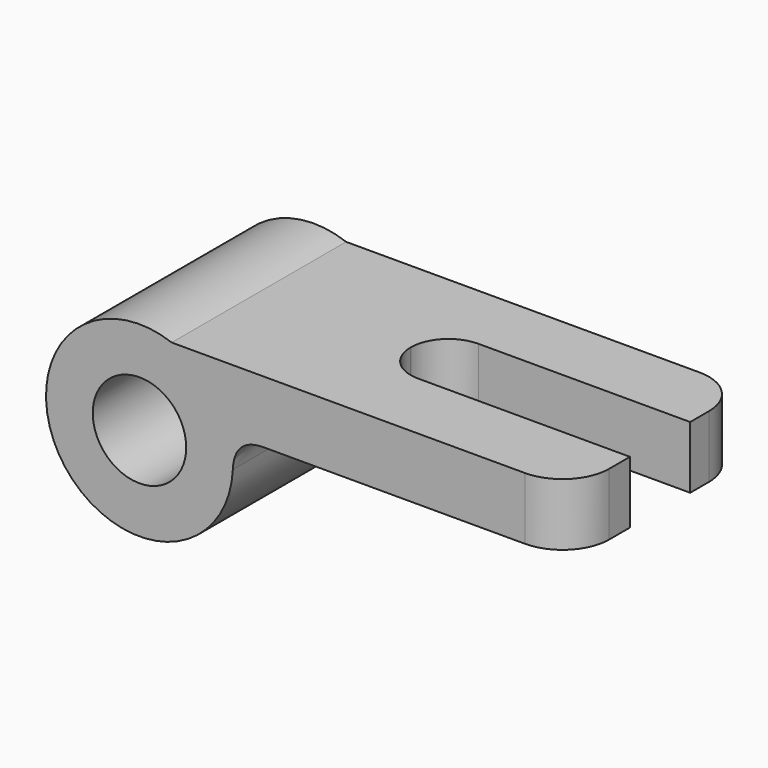
from build123d import *

# Parameters (mm, degrees)
F0_R        = 19.05
F1_DEPTH    = 44.45
F2_W        = 88.9
F2_H        = 12.7
F3_DEPTH    = 44.45
F4_T1_DEPTH = 44.45
F5_R        = 9.525
F6_DEPTH    = 44.45
F7_W        = 50.8
F7_H        = 15.3564938247
F8_DEPTH    = 12.7
F9_R        = 7.62
F10_R       = 7.62
F11_R       = 9.525
F12_R       = 9.525


# Not quite as in the source:
# - a fillet or chamfer that OpenCascade refuses, or shapes differently, is made with other operations: its cross-section is extruded or revolved along the edge and cut away or added


with BuildPart() as f1:
    # F0 (on Front) → F1 (new body)
    with BuildSketch(Plane.XZ):
        with Locations((-59.2879876494, 38.2781662047)):
            Circle(F0_R)
    extrude(amount=F1_DEPTH)

    # F2 (on Front) → F3 (join)
    with BuildSketch(Plane.XZ):
        with Locations((-15.6031847, 49.8112538493)):
            Rectangle(F2_W, F2_H)
    extrude(amount=F3_DEPTH)

    # F4: fillet of radius 6.35 on 1 edges, made by hand

    # F4_s2 → F4_t1 (join)
    with BuildSketch(Plane.XZ):
        with BuildLine():
            add(Edge.make_bspline(
                [(-40.2581018773, 37.4029819382), (-39.9794820095, 43.4612538493), (-33.91480662, 43.4612538493)],
                knots=[0, 0, 0, 1, 1, 1], degree=2, weights=[1, 1, 1]))
            Line((-33.91480662, 43.4612538493), (-40.9566455691, 43.4612538493))
            ThreePointArc((-40.9566455691, 43.4612538493), (-40.3633740127, 40.4602520649), (-40.2581018773, 37.4029819382))
        make_face()
    extrude(amount=F4_T1_DEPTH)

    # F5 (on face) → F6 (cut)
    with BuildSketch(Plane.XZ.offset(44.45)):
        with Locations((-59.2879876494, 38.2781662047)):
            Circle(F5_R)
    extrude(amount=-F6_DEPTH, mode=Mode.SUBTRACT)

    # F7 (on face) → F8 (cut)
    with BuildSketch(Plane(origin=(0, 0, 43.4612538493), x_dir=(1, 0, 0), z_dir=(0, 0, -1))):
        with Locations((3.4468153, 21.9657469124)):
            Rectangle(F7_W, F7_H)
    extrude(amount=-F8_DEPTH, mode=Mode.SUBTRACT)

    # F9
    f9_edges = [f1.edges().sort_by_distance(p)[0] for p in [
        (-21.953185, -29.643994, 49.811254),
    ]]
    fillet(f9_edges, radius=F9_R)

    # F10
    f10_edges = [f1.edges().sort_by_distance(p)[0] for p in [
        (-21.953185, -14.2875, 49.811254),
    ]]
    fillet(f10_edges, radius=F10_R)

    # F11
    f11_edges = [f1.edges().sort_by_distance(p)[0] for p in [
        (28.846815, 0, 49.811254),
    ]]
    fillet(f11_edges, radius=F11_R)

    # F12
    f12_edges = [f1.edges().sort_by_distance(p)[0] for p in [
        (28.846815, -44.45, 49.811254),
    ]]
    fillet(f12_edges, radius=F12_R)


solid = f1.part
